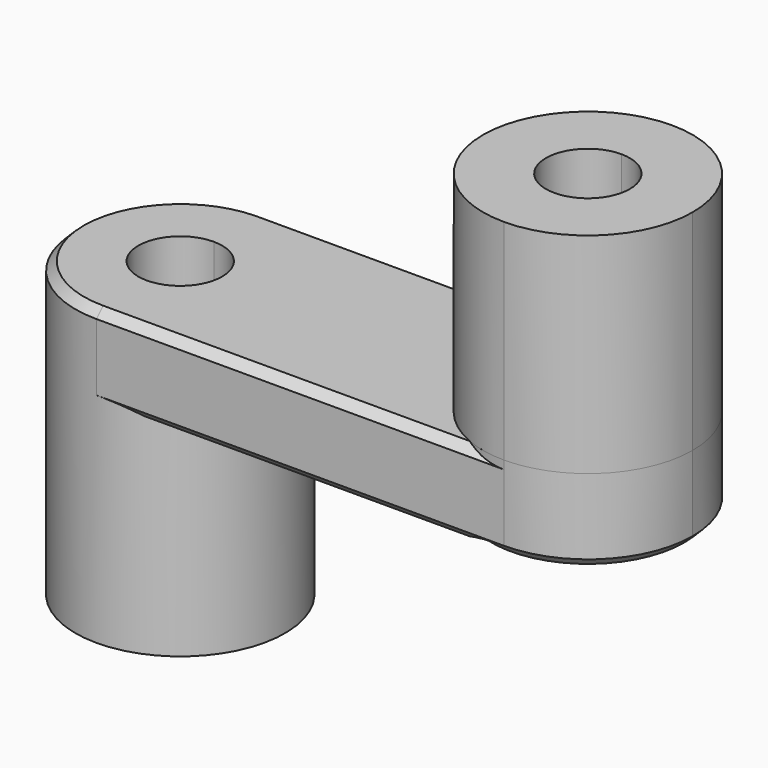
from build123d import *

# Parameters (mm, degrees)
F1_DEPTH     = 127
F2_DEPTH     = 177.8
F3_DEPTH     = 50.8
F4_DEPTH     = 50.8
F5_T1_DEPTH  = 286.1190739645
F5_T4_ANGLE  = 180
F5_T8_DEPTH  = 325.3115227011
F5_S9_R      = 63.5
F5_T10_DEPTH = 164
F5_T14_DEPTH = 325.3115227011
F5_S15_R     = 63.5
F5_T16_DEPTH = 164


# Not quite as in the source:
# - a fillet or chamfer that OpenCascade refuses, or shapes differently, is made with other operations: its cross-section is extruded or revolved along the edge and cut away or added


with BuildPart() as f1:
    # F0 (on Top) → F1 (new body)
    with BuildSketch(Plane.XY):
        with BuildLine():
            ThreePointArc((123.463312614, 63.5), (59.963312614, 0), (123.463312614, -63.5))
            Line((123.463312614, -63.5), (123.463312614, -25.4))
            ThreePointArc((123.463312614, -25.4), (98.063312614, 0), (123.463312614, 25.4))
            Line((123.463312614, 25.4), (123.463312614, 63.5))
        make_face()
        with BuildLine():
            Line((123.463312614, -25.4), (123.463312614, -63.5))
            ThreePointArc((123.463312614, -63.5), (168.3645932193, -44.9012806053), (186.963312614, 0))
            ThreePointArc((186.963312614, 0), (168.3645932193, 44.9012806053), (123.463312614, 63.5))
            Line((123.463312614, 63.5), (123.463312614, 25.4))
            ThreePointArc((123.463312614, 25.4), (141.4238248561, 17.9605122421), (148.863312614, 0))
            ThreePointArc((148.863312614, 0), (141.4238248561, -17.9605122421), (123.463312614, -25.4))
        make_face()
    extrude(amount=F1_DEPTH)



with BuildPart() as f2:
    # F0 (on Top) → F2 (new body)
    with BuildSketch(Plane.XY):
        with BuildLine():
            ThreePointArc((-123.463312614, 63.5), (-186.963312614, 0), (-123.463312614, -63.5))
            Line((-123.463312614, -63.5), (-123.463312614, -25.4))
            ThreePointArc((-123.463312614, -25.4), (-148.863312614, 0), (-123.463312614, 25.4))
            Line((-123.463312614, 25.4), (-123.463312614, 63.5))
        make_face()
        with BuildLine():
            Line((-123.463312614, -25.4), (-123.463312614, -63.5))
            ThreePointArc((-123.463312614, -63.5), (-78.5620320086, -44.9012806053), (-59.963312614, 0))
            ThreePointArc((-59.963312614, 0), (-78.5620320086, 44.9012806053), (-123.463312614, 63.5))
            Line((-123.463312614, 63.5), (-123.463312614, 25.4))
            ThreePointArc((-123.463312614, 25.4), (-105.5028003718, 17.9605122421), (-98.063312614, 0))
            ThreePointArc((-98.063312614, 0), (-105.5028003718, -17.9605122421), (-123.463312614, -25.4))
        make_face()
    extrude(amount=-F2_DEPTH)


with BuildPart() as f1_1:
    add(f1.part)

    add(f2.part)  # F3 merges F2
    # F0 (on Top) → F3 (join)
    with BuildSketch(Plane.XY):
        with BuildLine():
            Line((-123.463312614, -63.5), (123.463312614, -63.5))
            ThreePointArc((123.463312614, -63.5), (59.963312614, 0), (123.463312614, 63.5))
            Line((123.463312614, 63.5), (-123.463312614, 63.5))
            ThreePointArc((-123.463312614, 63.5), (-78.5620320086, 44.9012806053), (-59.963312614, 0))
            ThreePointArc((-59.963312614, 0), (-78.5620320086, -44.9012806053), (-123.463312614, -63.5))
        make_face()
    extrude(amount=-F3_DEPTH)

    # F5: chamfer of 5.08 on 3 edges, made by hand

    # F5_s2 → F5_t1 (cut)
    with BuildSketch(Plane.YZ.offset(-123.463312614)):
        Polygon((63.5, -5.08), (58.42, 0), (63.5, 0), align=None)
        Polygon((-63.5, -5.08), (-58.42, 0), (-63.5, 0), align=None)
    extrude(amount=F5_T1_DEPTH, mode=Mode.SUBTRACT)

    # F5_s3 → F5_t4 (revolve, cut)
    with BuildSketch(Plane.YZ.offset(-123.463312614)):
        Polygon((63.5, -5.08), (58.42, 0), (63.5, 0), align=None)
    revolve(axis=Axis((-123.463312614, 0, 0), (0, 0, 1)), revolution_arc=F5_T4_ANGLE, mode=Mode.SUBTRACT)


with BuildPart() as f4:
    # F0 (on Top) → F4 (new body)
    with BuildSketch(Plane.XY):
        with BuildLine():
            Line((123.463312614, -25.4), (123.463312614, -63.5))
            ThreePointArc((123.463312614, -63.5), (168.3645932193, -44.9012806053), (186.963312614, 0))
            ThreePointArc((186.963312614, 0), (168.3645932193, 44.9012806053), (123.463312614, 63.5))
            Line((123.463312614, 63.5), (123.463312614, 25.4))
            ThreePointArc((123.463312614, 25.4), (141.4238248561, 17.9605122421), (148.863312614, 0))
            ThreePointArc((148.863312614, 0), (141.4238248561, -17.9605122421), (123.463312614, -25.4))
        make_face()
        with BuildLine():
            ThreePointArc((123.463312614, 63.5), (59.963312614, 0), (123.463312614, -63.5))
            Line((123.463312614, -63.5), (123.463312614, -25.4))
            ThreePointArc((123.463312614, -25.4), (98.063312614, 0), (123.463312614, 25.4))
            Line((123.463312614, 25.4), (123.463312614, 63.5))
        make_face()
    extrude(amount=-F4_DEPTH)

    # F5#2: chamfer of 5.08 on 1 edges, made by hand

    # F5_2_s1 → F5_2_t2 (revolve, cut)
    with BuildSketch(Plane.XZ):
        Polygon((186.963312614, -45.72), (181.883312614, -50.8), (186.963312614, -50.8), align=None)
    revolve(axis=Axis((123.463312614, 0, -50.8), (0, 0, 1)), mode=Mode.SUBTRACT)


with BuildPart() as f5_tool6:
    # F5_s7 → F5_t8 (new body)
    with BuildSketch(Plane.YZ.offset(-162.6557613506)):
        Polygon((-63.5, -45.72), (-58.42, -50.8), (-63.5, -50.8), align=None)
    extrude(amount=F5_T8_DEPTH)

    # F5_s9 → F5_t10 (cut, symmetric)
    with BuildSketch(Plane.XY.offset(-48.3)):
        with Locations((-123.463312614, 0)):
            Circle(F5_S9_R)
    extrude(amount=F5_T10_DEPTH, both=True, mode=Mode.SUBTRACT)


with BuildPart() as f1_2:
    add(f1_1.part)

    # F5_t5: cut F5_tool6
    add(f5_tool6.part, mode=Mode.SUBTRACT)


with BuildPart() as f5_tool12:
    # F5_s13 → F5_t14 (new body)
    with BuildSketch(Plane.YZ.offset(162.6557613506)):
        Polygon((58.42, -50.8), (63.5, -45.72), (63.5, -50.8), align=None)
    extrude(amount=-F5_T14_DEPTH)

    # F5_s15 → F5_t16 (cut, symmetric)
    with BuildSketch(Plane.XY.offset(-48.3)):
        with Locations((-123.463312614, 0)):
            Circle(F5_S15_R)
    extrude(amount=F5_T16_DEPTH, both=True, mode=Mode.SUBTRACT)


with BuildPart() as f1_3:
    add(f1_2.part)

    # F5_t11: cut F5_tool12
    add(f5_tool12.part, mode=Mode.SUBTRACT)


solid = Compound([f4.part, f1_3.part])
